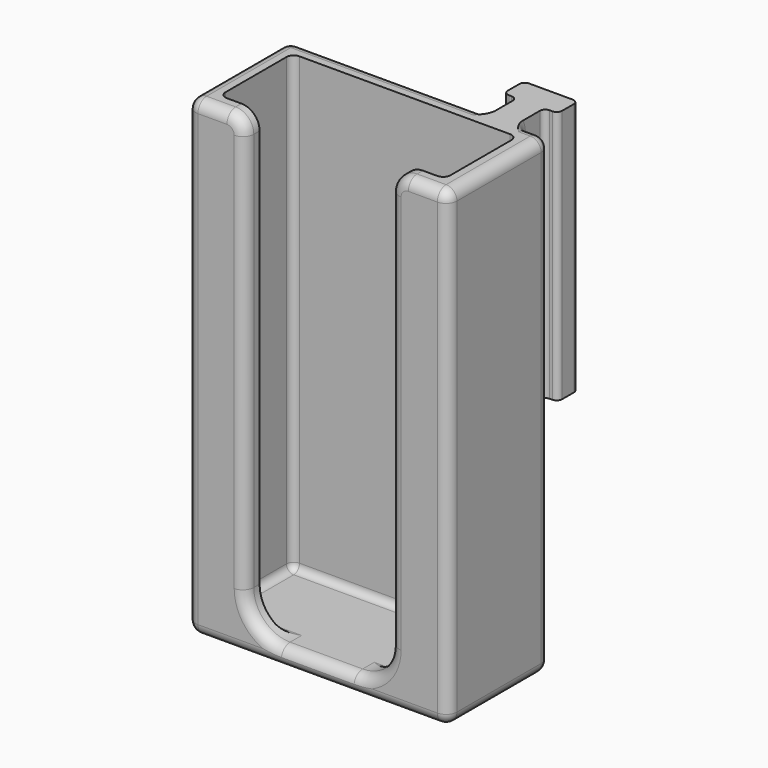
from build123d import *

# Parameters (mm, degrees)
F1_DEPTH      = 130
F2_W          = 15
F2_H          = 16
F3_DEPTH      = 60
F4_W          = 72
F4_H          = 35
F5_DEPTH      = 5
F6_R          = 10
F7_R          = 5
F8_R          = 3
F9_R          = 3
F10_R         = 2
F11_F1_R      = 2
F11_F2_R      = 2
F11_T3_DEPTH  = 123
F11_S7_W      = 2.04
F11_S7_H      = 2.04
F11_T8_DEPTH  = 2.04
F11_T11_DEPTH = 123
F11_S15_W     = 2.04
F11_S15_H     = 2.04
F11_T16_DEPTH = 2.04
F12_T1_DEPTH  = 124
F12_T3_DEPTH  = 20
F12_T5_DEPTH  = 66
F12_T7_DEPTH  = 8
F12_T9_DEPTH  = 110
F12_T11_DEPTH = 8
F12_T13_DEPTH = 52.75
F12_T15_DEPTH = 5.75
F12_T18_ANGLE = 90
F12_T20_ANGLE = 90
F12_T22_ANGLE = 90
F12_T24_ANGLE = 90
F12_T26_ANGLE = 90
F12_T28_ANGLE = 90
F12_T30_ANGLE = 90
F12_T32_ANGLE = 90
F12_T34_ANGLE = 90
F12_T36_ANGLE = 90
F12_T38_ANGLE = 90
F12_T40_ANGLE = 90
F13_T1_DEPTH  = 67
F13_T6_ANGLE  = 209.4141577086
F13_T12_ANGLE = 209.4141577086
F14_R         = 1.5
F15_R         = 1.5
F16_R         = 1.5


# Not quite as in the source:
# - a fillet or chamfer that OpenCascade refuses, or shapes differently, is made with other operations: its cross-section is extruded or revolved along the edge and cut away or added


with BuildPart() as f1:
    # F0 (on Top) → F1 (new body)
    with BuildSketch(Plane.XY):
        Polygon((-36, 17.5), (-36, -17.5), (-20, -17.5), (-20, -12.5000001863), (-30.9999994934, -12.5000001863), (-30.9999994934, 12.5), (30.9999994934, 12.5), (30.9999994934, -12.5000001863), (20, -12.5000001863), (20, -17.5), (36, -17.5), (36, 17.5), (27.25, 17.5), (27.25, 26.5), (31, 26.5), (31, 33.5), (23.5, 33.5), (16, 33.5), (16, 26.5), (19.75, 26.5), (19.75, 17.5), align=None)
    extrude(amount=F1_DEPTH)

    # F2 (on face) → F3 (cut)
    with BuildSketch(Plane(origin=(0, 0, 0), x_dir=(1, 0, 0), z_dir=(0, 0, -1))):
        with Locations((23.5, -25.5)):
            Rectangle(F2_W, F2_H)
    extrude(amount=-F3_DEPTH, mode=Mode.SUBTRACT)

    # F4 (on face) → F5 (join)
    with BuildSketch(Plane(origin=(0, 0, 0), x_dir=(1, 0, 0), z_dir=(0, 0, -1))):
        Rectangle(F4_W, F4_H)
    extrude(amount=-F5_DEPTH)

    # F6
    f6_edges = [f1.edges().sort_by_distance(p)[0] for p in [
        (-20, -15, 5),
        (20, -15, 5),
    ]]
    fillet(f6_edges, radius=F6_R)

    # F7
    f7_edges = [f1.edges().sort_by_distance(p)[0] for p in [
        (20, -15, 130),
        (-20, -15, 130),
    ]]
    fillet(f7_edges, radius=F7_R)

    # F8
    f8_edges = [f1.edges().sort_by_distance(p)[0] for p in [
        (36, 0, 130),
        (-36, 0, 130),
    ]]
    fillet(f8_edges, radius=F8_R)

    # F9
    f9_edges = [f1.edges().sort_by_distance(p)[0] for p in [
        (36, 0, 0),
        (-36, 0, 0),
    ]]
    fillet(f9_edges, radius=F9_R)

    # F10
    f10_edges = [f1.edges().sort_by_distance(p)[0] for p in [
        (30.999999, 0, 5),
        (0, 12.5, 5),
        (-30.999999, 0, 5),
    ]]
    fillet(f10_edges, radius=F10_R)

    # F11: fillet of radius 2 on 8 edges, made by hand

    # F11_f1
    f11_f1_edges = [f1.edges().sort_by_distance(p)[0] for p in [
        (24.4999997467, -12.5000001863, 5),
        (15, -12.5000001863, 5),
        (30.9999994934, -12.5000001863, 68.5),
        (30.4142130557, -12.5000001863, 5.5857864376),
    ]]
    fillet(f11_f1_edges, radius=F11_F1_R)

    # F11_f2
    f11_f2_edges = [f1.edges().sort_by_distance(p)[0] for p in [
        (-24.4999997467, -12.5000001863, 5),
        (-15, -12.5000001863, 5),
        (-30.4142130557, -12.5000001863, 5.5857864376),
        (-30.9999994934, -12.5000001863, 68.5),
    ]]
    fillet(f11_f2_edges, radius=F11_F2_R)

    # F11_s4 → F11_t3 (join)
    with BuildSketch(Plane.XY.offset(7)):
        with BuildLine():
            ThreePointArc((28.9999994934, 12.5), (30.4142130557, 11.9142135624), (30.9999994934, 10.5))
            Line((30.9999994934, 10.5), (31.0399994934, 10.5))
            Line((31.0399994934, 10.5), (31.0399994934, 12.54))
            Line((31.0399994934, 12.54), (28.9999994934, 12.54))
            Line((28.9999994934, 12.54), (28.9999994934, 12.5))
        make_face()
    extrude(amount=F11_T3_DEPTH)


with BuildPart() as f11_tool6:
    # F11_s7 → F11_t8 (new body)
    with BuildSketch(Plane.XZ.offset(-10.5)):
        with Locations((30.0199994934, 5.98)):
            Rectangle(F11_S7_W, F11_S7_H)
    extrude(amount=-F11_T8_DEPTH)

    # F11_s9 → F11_t10 (revolve, cut)
    with BuildSketch(Plane(origin=(28.9999994934, 10.5, 7), x_dir=(-0.7071067812, 0, 0.7071067812), z_dir=(-0.7071067812, 0, -0.7071067812))):
        with BuildLine():
            ThreePointArc((0, -2), (2, 0), (0, 2))
            Line((0, 2), (0, -2))
        make_face()
    revolve(axis=Axis((28.9999994934, 10.5, 7), (0, 1, 0)), mode=Mode.SUBTRACT)


with BuildPart() as f1_1:
    add(f1.part)

    # F11_t5: union F11_tool6
    add(f11_tool6.part)

    # F11_s12 → F11_t11 (join)
    with BuildSketch(Plane.XY.offset(7)):
        with BuildLine():
            ThreePointArc((-30.9999994934, 10.5), (-30.4142130557, 11.9142135624), (-28.9999994934, 12.5))
            Line((-28.9999994934, 12.5), (-28.9999994934, 12.54))
            Line((-28.9999994934, 12.54), (-31.0399994934, 12.54))
            Line((-31.0399994934, 12.54), (-31.0399994934, 10.5))
            Line((-31.0399994934, 10.5), (-30.9999994934, 10.5))
        make_face()
    extrude(amount=F11_T11_DEPTH)


with BuildPart() as f11_tool14:
    # F11_s15 → F11_t16 (new body)
    with BuildSketch(Plane.YZ.offset(-28.9999994934)):
        with Locations((11.52, 5.98)):
            Rectangle(F11_S15_W, F11_S15_H)
    extrude(amount=-F11_T16_DEPTH)

    # F11_s17 → F11_t18 (revolve, cut)
    with BuildSketch(Plane(origin=(-28.9999994934, 10.5, 7), x_dir=(0, -0.7071067812, 0.7071067812), z_dir=(0, -0.7071067812, -0.7071067812))):
        with BuildLine():
            ThreePointArc((0, -2), (2, 0), (0, 2))
            Line((0, 2), (0, -2))
        make_face()
    revolve(axis=Axis((-28.9999994934, 10.5, 7), (-1, 0, 0)), mode=Mode.SUBTRACT)


with BuildPart() as f1_2:
    add(f1_1.part)

    # F11_t13: union F11_tool14
    add(f11_tool14.part)

    # F12: fillet of radius 3 on 24 edges, made by hand

    # F12_s2 → F12_t1 (cut)
    with BuildSketch(Plane.XY.offset(3)):
        with BuildLine():
            ThreePointArc((33, -17.5), (35.1213203436, -16.6213203436), (36, -14.5))
            Line((36, -14.5), (36, -17.5))
            Line((36, -17.5), (33, -17.5))
        make_face()
        with BuildLine():
            ThreePointArc((-33, -17.5), (-35.1213203436, -16.6213203436), (-36, -14.5))
            Line((-36, -14.5), (-36, -17.5))
            Line((-36, -17.5), (-33, -17.5))
        make_face()
        with BuildLine():
            ThreePointArc((36, 14.5), (35.1213203436, 16.6213203436), (33, 17.5))
            Line((33, 17.5), (36, 17.5))
            Line((36, 17.5), (36, 14.5))
        make_face()
        with BuildLine():
            ThreePointArc((-36, 14.5), (-35.1213203436, 16.6213203436), (-33, 17.5))
            Line((-33, 17.5), (-36, 17.5))
            Line((-36, 17.5), (-36, 14.5))
        make_face()
    extrude(amount=F12_T1_DEPTH, mode=Mode.SUBTRACT)

    # F12_s4 → F12_t3 (cut)
    with BuildSketch(Plane.YZ.offset(-10)):
        with BuildLine():
            ThreePointArc((-14.5, 5), (-16.6213203436, 4.1213203436), (-17.5, 2))
            Line((-17.5, 2), (-17.5, 5))
            Line((-17.5, 5), (-14.5, 5))
        make_face()
    extrude(amount=F12_T3_DEPTH, mode=Mode.SUBTRACT)

    # F12_s6 → F12_t5 (cut)
    with BuildSketch(Plane.YZ.offset(-33)):
        with BuildLine():
            ThreePointArc((-17.5, 3), (-16.6213203436, 0.8786796564), (-14.5, 0))
            Line((-14.5, 0), (-17.5, 0))
            Line((-17.5, 0), (-17.5, 3))
        make_face()
        with BuildLine():
            ThreePointArc((14.5, 0), (16.6213203436, 0.8786796564), (17.5, 3))
            Line((17.5, 3), (17.5, 0))
            Line((17.5, 0), (14.5, 0))
        make_face()
    extrude(amount=F12_T5_DEPTH, mode=Mode.SUBTRACT)

    # F12_s8 → F12_t7 (cut)
    with BuildSketch(Plane.YZ.offset(-33)):
        with BuildLine():
            ThreePointArc((-17.5, 127), (-16.6213203436, 129.1213203436), (-14.5, 130))
            Line((-14.5, 130), (-17.5, 130))
            Line((-17.5, 130), (-17.5, 127))
        make_face()
    extrude(amount=F12_T7_DEPTH, mode=Mode.SUBTRACT)

    # F12_s10 → F12_t9 (cut)
    with BuildSketch(Plane.XY.offset(15)):
        with BuildLine():
            ThreePointArc((-23, -17.5), (-20.8786796564, -16.6213203436), (-20, -14.5))
            Line((-20, -14.5), (-20, -17.5))
            Line((-20, -17.5), (-23, -17.5))
        make_face()
        with BuildLine():
            ThreePointArc((23, -17.5), (20.8786796564, -16.6213203436), (20, -14.5))
            Line((20, -14.5), (20, -17.5))
            Line((20, -17.5), (23, -17.5))
        make_face()
    extrude(amount=F12_T9_DEPTH, mode=Mode.SUBTRACT)

    # F12_s12 → F12_t11 (cut)
    with BuildSketch(Plane.YZ.offset(25)):
        with BuildLine():
            ThreePointArc((-17.5, 127), (-16.6213203436, 129.1213203436), (-14.5, 130))
            Line((-14.5, 130), (-17.5, 130))
            Line((-17.5, 130), (-17.5, 127))
        make_face()
    extrude(amount=F12_T11_DEPTH, mode=Mode.SUBTRACT)

    # F12_s14 → F12_t13 (cut)
    with BuildSketch(Plane.YZ.offset(-33)):
        with BuildLine():
            ThreePointArc((14.5, 130), (16.6213203436, 129.1213203436), (17.5, 127))
            Line((17.5, 127), (17.5, 130))
            Line((17.5, 130), (14.5, 130))
        make_face()
    extrude(amount=F12_T13_DEPTH, mode=Mode.SUBTRACT)

    # F12_s16 → F12_t15 (cut)
    with BuildSketch(Plane.YZ.offset(27.25)):
        with BuildLine():
            ThreePointArc((14.5, 130), (16.6213203436, 129.1213203436), (17.5, 127))
            Line((17.5, 127), (17.5, 130))
            Line((17.5, 130), (14.5, 130))
        make_face()
    extrude(amount=F12_T15_DEPTH, mode=Mode.SUBTRACT)

    # F12_s17 → F12_t18 (revolve, cut)
    with BuildSketch(Plane.XY.offset(15)):
        with BuildLine():
            ThreePointArc((20, -14.5), (20.8786796564, -16.6213203436), (23, -17.5))
            Line((23, -17.5), (20, -17.5))
            Line((20, -17.5), (20, -14.5))
        make_face()
    revolve(axis=Axis((10, -17.5, 15), (0, 1, 0)), revolution_arc=F12_T18_ANGLE, mode=Mode.SUBTRACT)

    # F12_s19 → F12_t20 (revolve, cut)
    with BuildSketch(Plane.XY.offset(3)):
        with BuildLine():
            ThreePointArc((-33, -17.5), (-35.1213203436, -16.6213203436), (-36, -14.5))
            Line((-36, -14.5), (-36, -17.5))
            Line((-36, -17.5), (-33, -17.5))
        make_face()
    revolve(axis=Axis((-33, -17.5, 3), (0, -1, 0)), revolution_arc=F12_T20_ANGLE, mode=Mode.SUBTRACT)

    # F12_s21 → F12_t22 (revolve, cut)
    with BuildSketch(Plane.YZ.offset(-33)):
        with BuildLine():
            ThreePointArc((-17.5, 127), (-16.6213203436, 129.1213203436), (-14.5, 130))
            Line((-14.5, 130), (-17.5, 130))
            Line((-17.5, 130), (-17.5, 127))
        make_face()
    revolve(axis=Axis((-33, -17.5, 127), (0, -1, 0)), revolution_arc=F12_T22_ANGLE, mode=Mode.SUBTRACT)

    # F12_s23 → F12_t24 (revolve, cut)
    with BuildSketch(Plane.YZ.offset(33)):
        with BuildLine():
            ThreePointArc((-17.5, 3), (-16.6213203436, 0.8786796564), (-14.5, 0))
            Line((-14.5, 0), (-17.5, 0))
            Line((-17.5, 0), (-17.5, 3))
        make_face()
    revolve(axis=Axis((33, -17.5, 3), (0, -1, 0)), revolution_arc=F12_T24_ANGLE, mode=Mode.SUBTRACT)

    # F12_s25 → F12_t26 (revolve, cut)
    with BuildSketch(Plane.XY.offset(125)):
        with BuildLine():
            ThreePointArc((-23, -17.5), (-20.8786796564, -16.6213203436), (-20, -14.5))
            Line((-20, -14.5), (-20, -17.5))
            Line((-20, -17.5), (-23, -17.5))
        make_face()
    revolve(axis=Axis((-25, -17.5, 125), (0, -1, 0)), revolution_arc=F12_T26_ANGLE, mode=Mode.SUBTRACT)

    # F12_s27 → F12_t28 (revolve, cut)
    with BuildSketch(Plane.YZ.offset(33)):
        with BuildLine():
            ThreePointArc((-17.5, 127), (-16.6213203436, 129.1213203436), (-14.5, 130))
            Line((-14.5, 130), (-17.5, 130))
            Line((-17.5, 130), (-17.5, 127))
        make_face()
    revolve(axis=Axis((33, -17.5, 127), (0, 1, 0)), revolution_arc=F12_T28_ANGLE, mode=Mode.SUBTRACT)

    # F12_s29 → F12_t30 (revolve, cut)
    with BuildSketch(Plane.YZ.offset(-10)):
        with BuildLine():
            ThreePointArc((-17.5, 2), (-16.6213203436, 4.1213203436), (-14.5, 5))
            Line((-14.5, 5), (-17.5, 5))
            Line((-17.5, 5), (-17.5, 2))
        make_face()
    revolve(axis=Axis((-10, -17.5, 15), (0, 1, 0)), revolution_arc=F12_T30_ANGLE, mode=Mode.SUBTRACT)

    # F12_s31 → F12_t32 (revolve, cut)
    with BuildSketch(Plane.YZ.offset(25)):
        with BuildLine():
            ThreePointArc((-17.5, 127), (-16.6213203436, 129.1213203436), (-14.5, 130))
            Line((-14.5, 130), (-17.5, 130))
            Line((-17.5, 130), (-17.5, 127))
        make_face()
    revolve(axis=Axis((25, -17.5, 125), (0, -1, 0)), revolution_arc=F12_T32_ANGLE, mode=Mode.SUBTRACT)

    # F12_s33 → F12_t34 (revolve, cut)
    with BuildSketch(Plane.XY.offset(3)):
        with BuildLine():
            ThreePointArc((-36, 14.5), (-35.1213203436, 16.6213203436), (-33, 17.5))
            Line((-33, 17.5), (-36, 17.5))
            Line((-36, 17.5), (-36, 14.5))
        make_face()
    revolve(axis=Axis((-33, 17.5, 3), (0, -1, 0)), revolution_arc=F12_T34_ANGLE, mode=Mode.SUBTRACT)

    # F12_s35 → F12_t36 (revolve, cut)
    with BuildSketch(Plane.YZ.offset(-33)):
        with BuildLine():
            ThreePointArc((14.5, 130), (16.6213203436, 129.1213203436), (17.5, 127))
            Line((17.5, 127), (17.5, 130))
            Line((17.5, 130), (14.5, 130))
        make_face()
    revolve(axis=Axis((-33, 17.5, 127), (0, -1, 0)), revolution_arc=F12_T36_ANGLE, mode=Mode.SUBTRACT)

    # F12_s37 → F12_t38 (revolve, cut)
    with BuildSketch(Plane.YZ.offset(33)):
        with BuildLine():
            ThreePointArc((14.5, 0), (16.6213203436, 0.8786796564), (17.5, 3))
            Line((17.5, 3), (17.5, 0))
            Line((17.5, 0), (14.5, 0))
        make_face()
    revolve(axis=Axis((33, 17.5, 3), (0, -1, 0)), revolution_arc=F12_T38_ANGLE, mode=Mode.SUBTRACT)

    # F12_s39 → F12_t40 (revolve, cut)
    with BuildSketch(Plane.YZ.offset(33)):
        with BuildLine():
            ThreePointArc((14.5, 130), (16.6213203436, 129.1213203436), (17.5, 127))
            Line((17.5, 127), (17.5, 130))
            Line((17.5, 130), (14.5, 130))
        make_face()
    revolve(axis=Axis((33, 17.5, 127), (0, 1, 0)), revolution_arc=F12_T40_ANGLE, mode=Mode.SUBTRACT)

    # F13: fillet of radius 2.5 on 2 edges, made by hand

    # F13_s2 → F13_t1 (join)
    with BuildSketch(Plane.XY.offset(60)):
        with BuildLine():
            ThreePointArc((27.25, 20), (27.982233047, 18.232233047), (29.75, 17.5))
            Line((29.75, 17.5), (27.25, 17.5))
            Line((27.25, 17.5), (27.25, 20))
        make_face()
        with BuildLine():
            ThreePointArc((19.75, 20), (19.017766953, 18.232233047), (17.25, 17.5))
            Line((17.25, 17.5), (19.75, 17.5))
            Line((19.75, 17.5), (19.75, 20))
        make_face()
    extrude(amount=F13_T1_DEPTH)


with BuildPart() as f13_tool4:
    # F13_s5 → F13_t6 (revolve)
    with BuildSketch(Plane(origin=(0, -50.8345110114, 90.1646222656), x_dir=(1, 0, 0), z_dir=(0, 0.4911190143, -0.8710924829))):
        with BuildLine():
            ThreePointArc((19.75, -69.5029558217), (19.017766953, -71.2707227746), (17.25, -72.0029558217))
            Line((17.25, -72.0029558217), (19.75, -72.0029558217))
            Line((19.75, -72.0029558217), (19.75, -69.5029558217))
        make_face()
    revolve(axis=Axis((19.75, 14.5000000001, 127.0000000001), (-1, 0, 0)), revolution_arc=F13_T6_ANGLE)

    split(bisect_by=Plane.XZ.offset(-12.5), keep=Keep.BOTTOM)

    split(bisect_by=Plane.XY.offset(130), keep=Keep.BOTTOM)


with BuildPart() as f1_3:
    add(f1_2.part)

    # F13_t3: union F13_tool4
    add(f13_tool4.part)


with BuildPart() as f13_tool10:
    # F13_s11 → F13_t12 (revolve)
    with BuildSketch(Plane(origin=(0, -50.8345110114, 90.1646222656), x_dir=(1, 0, 0), z_dir=(0, 0.4911190143, -0.8710924829))):
        with BuildLine():
            ThreePointArc((29.75, -72.0029558217), (27.982233047, -71.2707227746), (27.25, -69.5029558217))
            Line((27.25, -69.5029558217), (27.25, -72.0029558217))
            Line((27.25, -72.0029558217), (29.75, -72.0029558217))
        make_face()
    revolve(axis=Axis((27.25, 14.5000000001, 127.0000000001), (-1, 0, 0)), revolution_arc=F13_T12_ANGLE)

    split(bisect_by=Plane.XZ.offset(-12.5), keep=Keep.BOTTOM)

    split(bisect_by=Plane.XY.offset(130), keep=Keep.BOTTOM)


with BuildPart() as f1_4:
    add(f1_3.part)

    # F13_t9: union F13_tool10
    add(f13_tool10.part)

    # F14
    f14_edges = [f1_4.edges().sort_by_distance(p)[0] for p in [
        (19.75, 26.5, 95),
        (27.25, 26.5, 95),
    ]]
    fillet(f14_edges, radius=F14_R)

    # F15
    f15_edges = [f1_4.edges().sort_by_distance(p)[0] for p in [
        (31, 33.5, 95),
        (16, 33.5, 95),
    ]]
    fillet(f15_edges, radius=F15_R)

    # F16
    f16_edges = [f1_4.edges().sort_by_distance(p)[0] for p in [
        (31, 26.5, 95),
        (16, 26.5, 95),
    ]]
    fillet(f16_edges, radius=F16_R)


solid = f1_4.part
